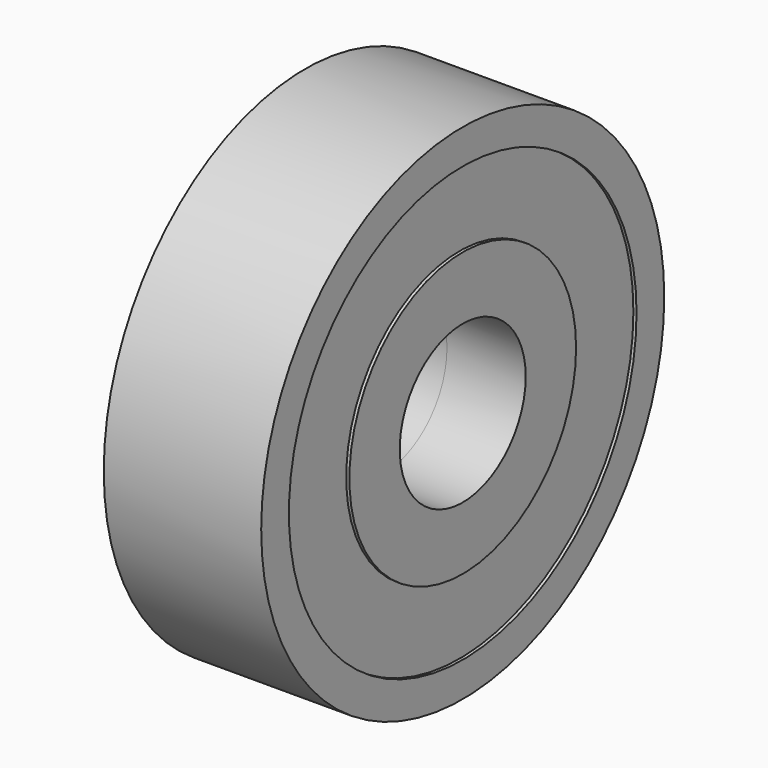
from build123d import *

# Parameters (mm, degrees)
F0_R          = 8
F0_R_2        = 2.5
F1_DEPTH      = 2.5
F1_DEPTH_BACK = 2.5
F2_R          = 6.9
F2_R_2        = 4.5
F3_DEPTH      = 0.1


# Not quite as in the source:
# - a pattern or mirror of a feature is missing from the dataset's text; its kind, count and spacing are read off the source's solid


with BuildPart() as f1:
    # F0 (on Right) → F1 (new body, two sides)
    with BuildSketch(Plane.YZ) as f1_sk:
        Circle(F0_R)
        Circle(F0_R_2, mode=Mode.SUBTRACT)
    extrude(amount=F1_DEPTH)
    extrude(f1_sk.sketch, amount=-F1_DEPTH_BACK)

    # F2 (on face) → F3 (cut)
    with BuildSketch(Plane.YZ.offset(2.5)):
        Circle(F2_R)
        Circle(F2_R_2, mode=Mode.SUBTRACT)
    f3 = extrude(amount=-F3_DEPTH, mode=Mode.SUBTRACT)

    # F3_copies: F3 across plane
    add(f3.mirror(Plane(origin=(0, 0, 0), x_dir=(0, 0, -1), z_dir=(-1, 0, 0))), mode=Mode.SUBTRACT)


solid = f1.part
